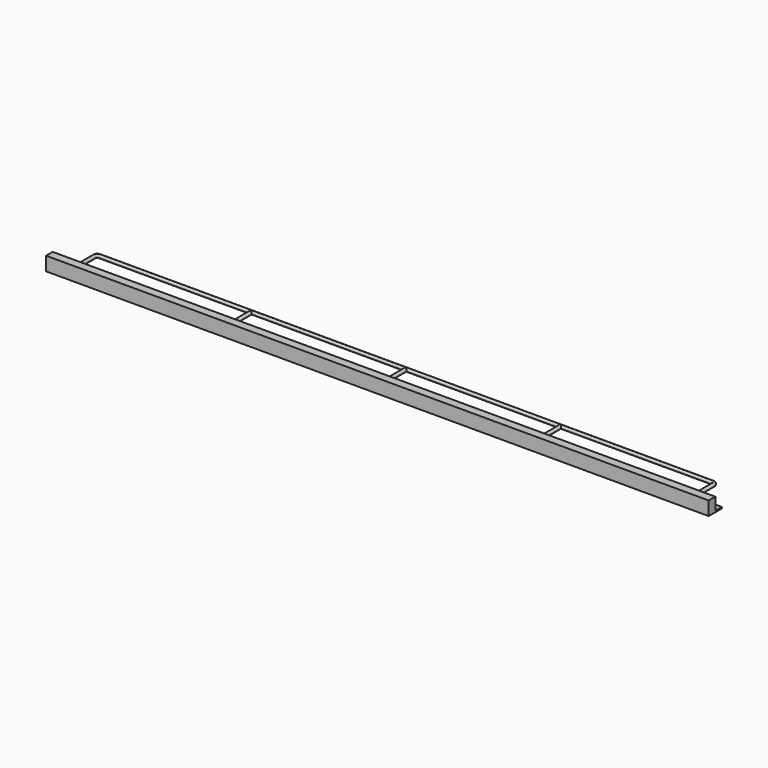
from build123d import *

# Parameters (mm, degrees)
F0_W          = 2405
F0_H          = 50
F1_DEPTH      = 15
F1_DEPTH_BACK = 15
F2_W          = 60
F2_H          = 30
F3_DEPTH      = 5
F4_W          = 60
F4_H          = 30
F5_DEPTH      = 5
F6_R          = 6
F7_DEPTH      = 5
F9_DEPTH      = 5
F10_DEPTH     = 5
F11_DEPTH     = 5


# Not quite as in the source:
# - a feature of the source that left no trace in its solid (it failed there, or was rolled back) is left out
# - a pattern or mirror of a feature is missing from the dataset's text; its kind, count and spacing are read off the source's solid
# - a feature names something its author has since deleted; it is built from what else it names


with BuildPart() as f1:
    # F0 (on Front) → F1 (new body, two sides)
    with BuildSketch(Plane.XZ) as f1_sk:
        Rectangle(F0_W, F0_H)
    extrude(amount=F1_DEPTH)
    extrude(f1_sk.sketch, amount=-F1_DEPTH_BACK)

    # F2 (on face) → F3 (join)
    with BuildSketch(Plane(origin=(0, 0, -25), x_dir=(1, 0, 0), z_dir=(0, 0, -1))):
        with Locations((-1172.5, -30)):
            Rectangle(F2_W, F2_H)
        Polygon((-1142.5, 15), (-1202.5, 15), (-1202.5, 0), (-1202.5, -15), (-1142.5, -15), align=None)
    extrude(amount=F3_DEPTH)

    # F4 (on face) → F5 (join)
    with BuildSketch(Plane(origin=(0, 0, -25), x_dir=(1, 0, 0), z_dir=(0, 0, -1))):
        with Locations((1172.5, -30)):
            Rectangle(F4_W, F4_H)
        Polygon((1202.5, 0), (1202.5, 15), (1142.5, 15), (1142.5, -15), (1202.5, -15), align=None)
    extrude(amount=F5_DEPTH)

    # F6 (on face) → F7 (cut, through all)
    with BuildSketch(Plane(origin=(0, 0, -30), x_dir=(1, 0, 0), z_dir=(0, 0, -1))):
        with Locations((1167.5, -30)):
            Circle(F6_R)
    extrude(amount=-F7_DEPTH, mode=Mode.SUBTRACT)

    # F8 (on face) → F9 (cut, through all)
    with BuildSketch(Plane(origin=(0, 0, -30), x_dir=(1, 0, 0), z_dir=(0, 0, -1))):
        with BuildLine():
            ThreePointArc((-1173.5, -30), (-1167.5, -36), (-1161.5, -30))
            ThreePointArc((-1161.5, -30), (-1167.5, -24), (-1173.5, -30))
        make_face()
    extrude(amount=-F9_DEPTH, mode=Mode.SUBTRACT)

    # F10 (add): faces of the model
    f10_faces = [f1.faces().sort_by_distance(p)[0] for p in [
        (1172.5, 44.3291796068, -25),
        (-1201.8291796068, 30, -25),
    ]]
    extrude(f10_faces, amount=F10_DEPTH)

    # F11 (cut): faces of the model
    f11_faces = [f1.faces().sort_by_distance(p)[0] for p in [
        (-1172.6621744947, 14.5134765159, -30),
        (1172.6621744947, 14.5134765159, -30),
    ]]
    extrude(f11_faces, amount=-F11_DEPTH, mode=Mode.SUBTRACT)

    # F14: sweep along a path in F13
    with BuildLine(Plane.XY) as f14_path:
        Line((1122.5, 15), (1122.5, 105))
        ThreePointArc((1122.5, 105), (1119.5710678119, 112.0710678119), (1112.5, 115))
        Line((1112.5, 115), (-1112.5, 115))
        ThreePointArc((-1112.5, 115), (-1119.5710678119, 112.0710678119), (-1122.5, 105))
        Line((-1122.5, 105), (-1122.5, 15))
    # F12 (on face) → F14 (sweep)
    with BuildSketch(Plane(origin=(0, 15, 0), x_dir=(-1, 0, 0), z_dir=(0, 1, 0))):
        with BuildLine():
            Line((-1122.5, 0), (-1122.5, 6))
            ThreePointArc((-1122.5, 6), (-1126.7426406871, -4.2426406871), (-1116.5, 0))
            Line((-1116.5, 0), (-1122.5, 0))
        make_face()
        with BuildLine():
            ThreePointArc((-1116.5, 0), (-1118.2573593129, 4.2426406871), (-1122.5, 6))
            Line((-1122.5, 6), (-1122.5, 0))
            Line((-1122.5, 0), (-1116.5, 0))
        make_face()
    sweep(path=f14_path.line)

    # F15: sweep along a path in F13
    with BuildLine(Plane.XY) as f15_path:
        Line((-561.25, 115), (-561.25, 15))
    # F12 (on face) → F15 (sweep)
    with BuildSketch(Plane(origin=(0, 15, 0), x_dir=(-1, 0, 0), z_dir=(0, 1, 0))):
        with BuildLine():
            ThreePointArc((567.25, 0), (561.25, 6), (555.25, 0))
            Line((555.25, 0), (567.25, 0))
        make_face()
        with BuildLine():
            Line((567.25, 0), (555.25, 0))
            ThreePointArc((555.25, 0), (561.25, -6), (567.25, 0))
        make_face()
    f15 = sweep(path=f15_path.line)

    # F15_copies: F15 across plane
    add(f15.mirror(Plane(origin=(-280.625, 0, 0), x_dir=(0, 0, 1), z_dir=(1, 0, 0))))

    # F17: sweep along a path in F13
    with BuildLine(Plane.XY) as f17_path:
        Line((561.25, 115), (561.25, 15))
    # F12 (on face) → F17 (sweep)
    with BuildSketch(Plane(origin=(0, 15, 0), x_dir=(-1, 0, 0), z_dir=(0, 1, 0))):
        with BuildLine():
            ThreePointArc((-555.25, 0), (-561.25, 6), (-567.25, 0))
            Line((-567.25, 0), (-555.25, 0))
        make_face()
        with BuildLine():
            Line((-555.25, 0), (-567.25, 0))
            ThreePointArc((-567.25, 0), (-561.25, -6), (-555.25, 0))
        make_face()
    sweep(path=f17_path.line)


solid = f1.part
